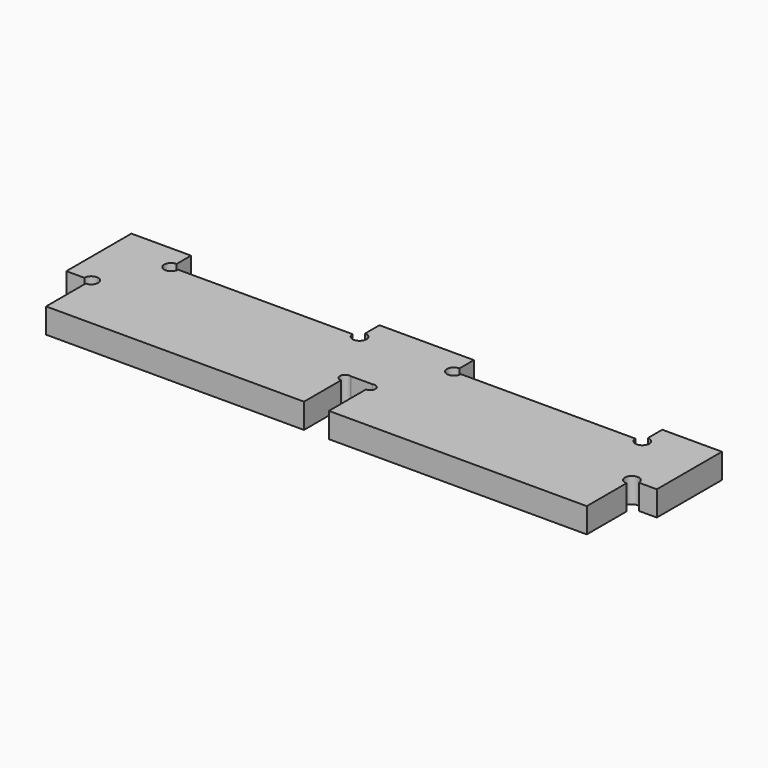
from build123d import *

# Parameters (mm, degrees)
F1_W      = 431.8
F1_H      = 82.55
F2_DEPTH  = 18.2118
F4_DEPTH  = 18.2128
F6_DEPTH  = 18.2128
F7_W      = 18.2118
F7_H      = 18.2118
F7_W_2    = 25.4
F8_DEPTH  = 18.2118
F9_R      = 5.08
F10_DEPTH = 18.2128


# Not quite as in the source:
# - a variable given as a bare number and used for a length is read in inches; the dataset says mm whatever the document's units were
# - a feature names something its author has since deleted; it is built from what else it names


with BuildPart() as f2:
    # F1 (on Top) → F2 (new body)
    with BuildSketch(Plane.XY):
        Rectangle(F1_W, F1_H)
    extrude(amount=F2_DEPTH)

    # F3 (on face) → F4 (cut, through all)
    with BuildSketch(Plane.XY.offset(18.2118)):
        Polygon((-215.9, 0), (-215.9, -41.275), (-197.6882, -41.275), (-197.6882, -5.08), (-197.6882, 0), (-202.7682, 0), align=None)
        with BuildLine():
            Line((-197.6882, 0), (-197.6882, -5.08))
            ThreePointArc((-197.6882, -5.08), (-194.0960975516, 3.5921024484), (-202.7682, 0))
            Line((-202.7682, 0), (-197.6882, 0))
        make_face()
        with BuildLine():
            Line((197.6882, 0), (202.7682, 0))
            ThreePointArc((202.7682, 0), (194.0960975516, 3.5921024484), (197.6882, -5.08))
            Line((197.6882, -5.08), (197.6882, 0))
        make_face()
        Polygon((197.6882, -5.08), (197.6882, -41.275), (215.9, -41.275), (215.9, 0), (202.7682, 0), (197.6882, 0), align=None)
    extrude(amount=-F4_DEPTH, mode=Mode.SUBTRACT)

    # F5 (on face) → F6 (cut, through all)
    with BuildSketch(Plane.XY.offset(18.2118)):
        Polygon((-9.1059, -7.4021024484), (-9.1059, -41.275), (9.1059, -41.275), (9.1059, -7.4021024484), (9.1059, 0), (7.8359, 0), (-7.8359, 0), (-9.1059, 0), align=None)
        with BuildLine():
            ThreePointArc((-7.8359, 0), (-12.8610305123, -2.9478239095), (-9.1059, -7.4021024484))
            Line((-9.1059, -7.4021024484), (-9.1059, 0))
            Line((-9.1059, 0), (-7.8359, 0))
        make_face()
        with BuildLine():
            Line((9.1059, 0), (9.1059, -7.4021024484))
            ThreePointArc((9.1059, -7.4021024484), (12.8610305123, -2.9478239095), (7.8359, 0))
            Line((7.8359, 0), (9.1059, 0))
        make_face()
    extrude(amount=-F6_DEPTH, mode=Mode.SUBTRACT)

    # F7 (on face) → F8 (join)
    with BuildSketch(Plane(origin=(0, 41.275, 0), x_dir=(-1, 0, 0), z_dir=(0, 1, 0))):
        with Locations((0, 9.1059)):
            Rectangle(F7_W, F7_H)
        with Locations((-21.8059, 9.1059)):
            Rectangle(F7_W_2, F7_H)
        with Locations((21.8059, 9.1059)):
            Rectangle(F7_W_2, F7_H)
        with Locations((-206.7941, 9.1059)):
            Rectangle(F7_W, F7_H)
        with Locations((-184.9882, 9.1059)):
            Rectangle(F7_W_2, F7_H)
        with Locations((184.9882, 9.1059)):
            Rectangle(F7_W_2, F7_H)
        with Locations((206.7941, 9.1059)):
            Rectangle(F7_W, F7_H)
    extrude(amount=F8_DEPTH)

    # F9 (on face) → F10 (cut, through all)
    with BuildSketch(Plane(origin=(0, 0, 0), x_dir=(1, 0, 0), z_dir=(0, 0, -1))):
        with Locations((34.5059, -41.275)):
            Circle(F9_R)
        with Locations((-34.5059, -41.275)):
            Circle(F9_R)
        with Locations((172.2882, -41.275)):
            Circle(F9_R)
        with Locations((-172.2882, -41.275)):
            Circle(F9_R)
    extrude(amount=-F10_DEPTH, mode=Mode.SUBTRACT)


solid = f2.part
